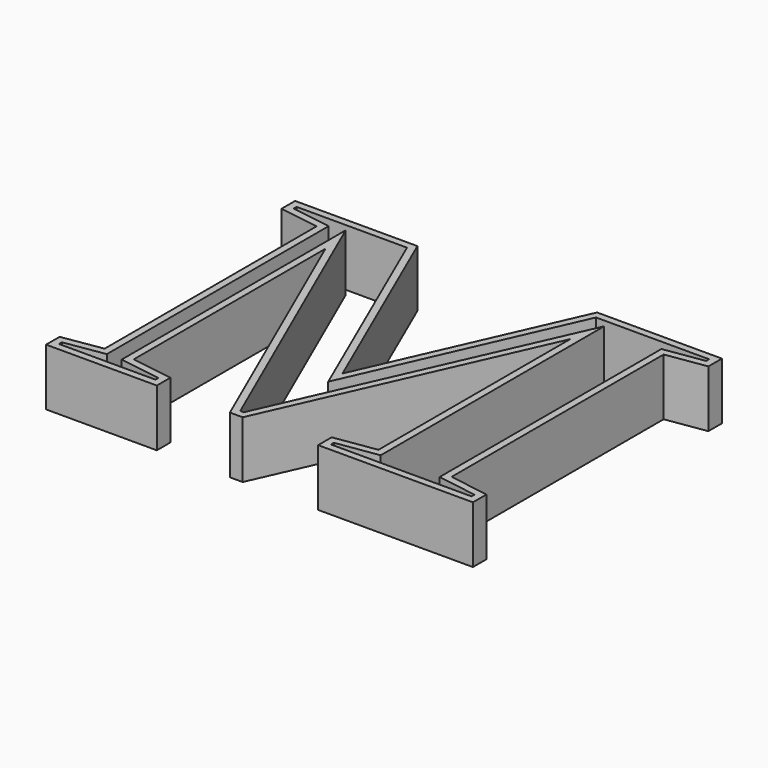
from build123d import *

# Parameters (mm, degrees)
F0_TEXT_SIZE = 166.6666666667
F1_DEPTH     = 20
F2_T         = -2.5
F3_DEPTH     = 25


# Not quite as in the source:
# - Text() gives the source's letters only with a copy of the font that has no kerning and outlines rounded to 1/6400 em; it was checked with that copy


with BuildPart() as f1:
    # F0 (on Top) → F1 (new body)
    with BuildSketch(Plane.XY):
        with Locations((-81.4583333333, -60)):
            Text('M', F0_TEXT_SIZE, font='Tinos', font_style=FontStyle.BOLD, text_align=(TextAlign.LEFT, TextAlign.BOTTOM))
    extrude(amount=F1_DEPTH)

    # F2
    f2_openings = [f1.faces().sort_by_distance(p)[0] for p in [
        (-56.279385, -9.817708, 20),
    ]]
    offset(amount=F2_T, openings=f2_openings, kind=Kind.INTERSECTION)

    # F3 (cut): a face of the model
    f3_faces = [f1.faces().sort_by_distance(p)[0] for p in [
        (-49.8759349976, -56.8684796131, 2.5),
    ]]
    extrude(f3_faces, amount=-F3_DEPTH, mode=Mode.SUBTRACT)


solid = f1.part
